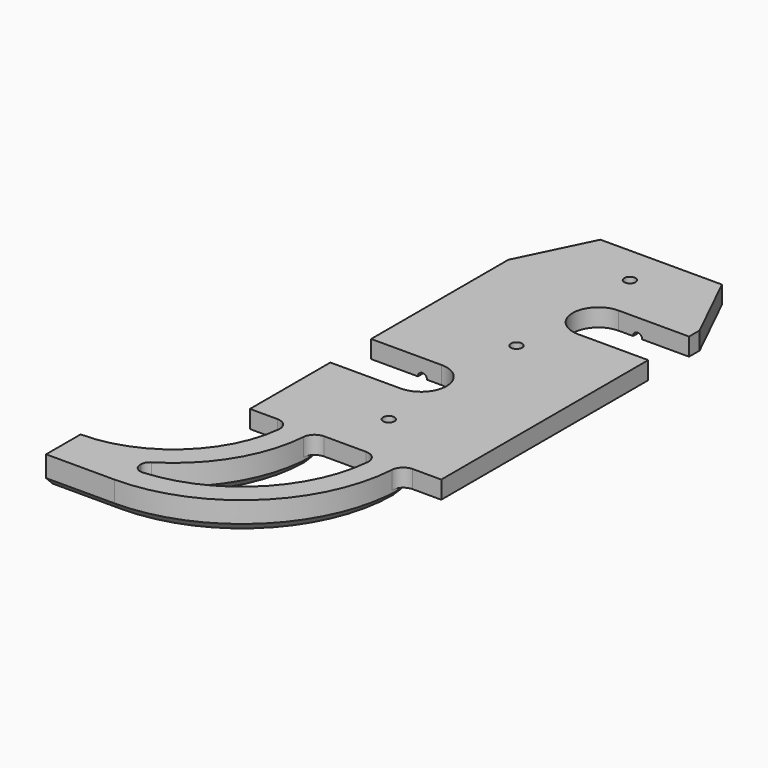
from build123d import *

# Parameters (mm, degrees)
F1_DEPTH       = 4.953
F3_DEPTH       = 4.954
F5_DEPTH       = 109.983
F7_DEPTH       = 15.494
F8_W           = 74.6252
F8_H           = 44.45
F9_DEPTH       = 4.953
F9_DEPTH_BACK  = 3.175
F11_R          = 1.27
F17_DEPTH      = 3.176
F17_DEPTH_BACK = 4.954
F19_D          = 3.15
F20_R          = 3.302
F21_R          = 2.5393938838
F22_SIZE       = 2.286


# Not quite as in the source:
# - a feature names something its author has since deleted; it is built from what else it names


with BuildPart() as f1:
    # F0 (on Top) → F1 (new body)
    with BuildSketch(Plane.XY):
        Polygon((-26.67, 0), (26.67, 0), (26.67, 90.043), (16.9418, 109.982), (-16.9418, 109.982), (-26.67, 90.043), align=None)
    extrude(amount=F1_DEPTH)

    # F2 (on Top) → F3 (cut, through all)
    with BuildSketch(Plane.XY):
        with BuildLine():
            Line((-26.67, 28.0162), (-7.0612, 28.0162))
            ThreePointArc((-7.0612, 28.0162), (0.0508, 35.1282), (-7.0612, 42.2402))
            Line((-7.0612, 42.2402), (-26.67, 42.2402))
            Line((-26.67, 42.2402), (-26.67, 28.0162))
        make_face()
        with BuildLine():
            Line((26.67, 86.36), (7.0612, 86.36))
            ThreePointArc((7.0612, 86.36), (-0.0508, 79.248), (7.0612, 72.136))
            Line((7.0612, 72.136), (26.67, 72.136))
            Line((26.67, 72.136), (26.67, 86.36))
        make_face()
    extrude(amount=F3_DEPTH, mode=Mode.SUBTRACT)

    # F4 (on face) → F5 (cut, through all)
    with BuildSketch(Plane.XZ):
        with BuildLine():
            ThreePointArc((-11.0871, 0), (-12.3571, 1.27), (-13.6271, 0))
            Line((-13.6271, 0), (-11.0871, 0))
        make_face()
        with BuildLine():
            ThreePointArc((13.6271, 0), (12.3571, 1.27), (11.0871, 0))
            Line((11.0871, 0), (13.6271, 0))
        make_face()
    extrude(amount=-F5_DEPTH, mode=Mode.SUBTRACT)

    # F6 (on face) → F7 (cut)
    with BuildSketch(Plane(origin=(0, 109.982, 0), x_dir=(-1, 0, 0), z_dir=(0, 1, 0))):
        with BuildLine():
            ThreePointArc((-9.2837, 0), (-12.3571, 3.0734), (-15.4305, 0))
            Line((-15.4305, 0), (-9.2837, 0))
        make_face()
        with BuildLine():
            ThreePointArc((15.4305, 0), (12.3571, 3.0734), (9.2837, 0))
            Line((9.2837, 0), (15.4305, 0))
        make_face()
    extrude(amount=-F7_DEPTH, mode=Mode.SUBTRACT)

    # F8 (on Top) → F9 (join, two sides)
    with BuildSketch(Plane.XY) as f9_sk:
        with Locations((-10.6426, -22.225)):
            Rectangle(F8_W, F8_H)
    extrude(amount=F9_DEPTH)
    extrude(f9_sk.sketch, amount=-F9_DEPTH_BACK)

    # F12: sweep along a path in F10
    with BuildLine(Plane.XY) as f12_path:
        Line((-47.9552, -41.275), (-28.9179, -41.275))
        ThreePointArc((-28.9179, -41.275), (0.2679323935, -29.1858323935), (12.3571, 0))
    # F11 (on face) → F12 (sweep, cut)
    with BuildSketch(Plane(origin=(0, 0, 0), x_dir=(-1, 0, 0), z_dir=(0, 1, 0))):
        with Locations((-12.3571, 0)):
            Circle(F11_R)
    sweep(path=f12_path.line, mode=Mode.SUBTRACT)

    # F15: sweep along a path in F13
    with BuildLine(Plane.XY) as f15_path:
        ThreePointArc((-12.3571, 0), (-22.7835420926, -25.1716579074), (-47.9552, -35.5981))
    # F14 (on face) → F15 (sweep, cut)
    with BuildSketch(Plane(origin=(0, 0, 0), x_dir=(-1, 0, 0), z_dir=(0, 1, 0))):
        with BuildLine():
            ThreePointArc((11.0871, 0), (12.3571, -1.27), (13.6271, 0))
            ThreePointArc((13.6271, 0), (12.3571, 1.27), (11.0871, 0))
        make_face()
    sweep(path=f15_path.line, mode=Mode.SUBTRACT)

    # F16 (on Top) → F17 (cut, two sides)
    with BuildSketch(Plane.XY) as f17_sk:
        with BuildLine():
            Line((-28.9179, -44.45), (26.67, -44.45))
            Line((26.67, -44.45), (26.67, 0))
            Line((26.67, 0), (15.5321, 0))
            ThreePointArc((15.5321, 0), (2.5129964237, -31.4308964237), (-28.9179, -44.45))
        make_face()
        with BuildLine():
            ThreePointArc((-28.9179, -38.1), (-1.9771316368, -26.9407683632), (9.1821, 0))
            Line((9.1821, 0), (-9.1821, 0))
            ThreePointArc((-9.1821, 0), (-14.4660215428, -19.5404250178), (-28.8776213731, -33.7549889252))
            Line((-28.8776213731, -33.7549889252), (-28.9179, -38.1))
        make_face()
        with BuildLine():
            ThreePointArc((-47.9552, -32.4231), (-25.0286061229, -22.9265938771), (-15.5321, 0))
            Line((-15.5321, 0), (-47.9552, 0))
            Line((-47.9552, 0), (-47.9552, -32.4231))
        make_face()
    extrude(amount=-F17_DEPTH, mode=Mode.SUBTRACT)
    extrude(f17_sk.sketch, amount=F17_DEPTH_BACK, mode=Mode.SUBTRACT)

    # F19 (through all)
    with Locations(Plane.XY.offset(4.953)):
        with Locations((0, 99.1108), (0, 59.563), (0, 15.0622)):
            Hole(F19_D / 2)

    # F20
    f20_edges = [f1.edges().sort_by_distance(p)[0] for p in [
        (9.1821, 0, 2.4765),
        (-9.1821, 0, 2.4765),
        (15.5321, 0, 2.4765),
        (-15.5321, 0, 2.4765),
    ]]
    fillet(f20_edges, radius=F20_R)

    # F21
    f21_edges = [f1.edges().sort_by_distance(p)[0] for p in [
        (-28.877621, -33.754989, 0.889),
        (-28.9179, -38.1, 0.889),
    ]]
    fillet(f21_edges, radius=F21_R)

    # F22
    f22_edges = [f1.edges().sort_by_distance(p)[0] for p in [
        (-38.43655, -44.45, -3.175),
        (-14.121028, -18.936792, -3.175),
        (-28.561794, -33.963255, -3.175),
        (-28.892105, -35.317366, -3.175),
        (-28.092277, -37.319249, -3.175),
        (-1.022826, -25.951394, -3.175),
        (-25.028606, -22.926594, -3.175),
        (2.512996, -31.430896, -3.175),
    ]]
    chamfer(f22_edges, length=F22_SIZE)


solid = f1.part
